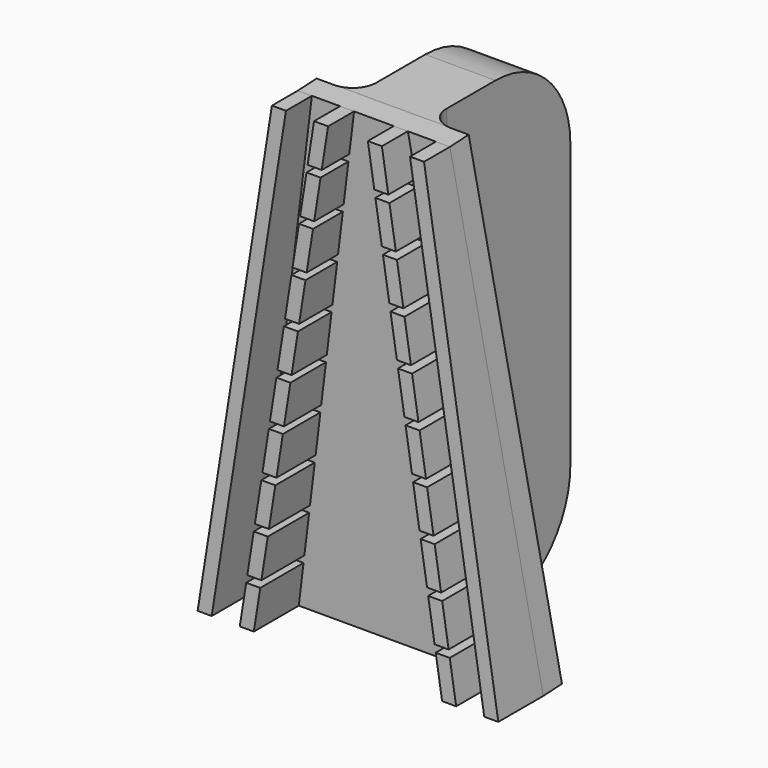
from build123d import *

# Parameters (mm, degrees)
F1_DEPTH     = 12
F3_DEPTH     = 40
F5_DEPTH     = 5
F6_W         = 38
F6_H         = 100.4237157875
F7_DEPTH     = 7.5
F9_DEPTH     = 7.5
F10_T4_DEPTH = 100.2951088773
F10_T9_DEPTH = 100.2951088773
F11_R        = 20


# Not quite as in the source:
# - a fillet or chamfer that OpenCascade refuses, or shapes differently, is made with other operations: its cross-section is extruded or revolved along the edge and cut away or added


with BuildPart() as f1:
    # F0 (on Front) → F1 (new body)
    with BuildSketch(Plane.XZ):
        Polygon((-18.7375766605, 8.6666666667), (-21.7375766605, 8.6666666667), (-23.11024181, 0), (-20.11024181, 0), align=None)
    extrude(amount=F1_DEPTH)


with BuildPart() as f1b:
    # F0 (on Front) → F1, piece 2 (new body)
    with BuildSketch(Plane.XZ):
        Polygon((21.7375766605, 8.6666666667), (18.7375766605, 8.6666666667), (20.11024181, 0), (23.11024181, 0), align=None)
    extrude(amount=F1_DEPTH)


with BuildPart() as f1c:
    # F0 (on Front) → F1, piece 3 (new body)
    with BuildSketch(Plane.XZ):
        Polygon((-20.1273348505, 18.8333333333), (-21.5, 10.1666666667), (-18.5, 10.1666666667), (-17.1273348505, 18.8333333333), align=None)
    extrude(amount=F1_DEPTH)


with BuildPart() as f1d:
    # F0 (on Front) → F1, piece 4 (new body)
    with BuildSketch(Plane.XZ):
        Polygon((17.1273348505, 18.8333333333), (18.5, 10.1666666667), (21.5, 10.1666666667), (20.1273348505, 18.8333333333), align=None)
    extrude(amount=F1_DEPTH)


with BuildPart() as f1e:
    # F0 (on Front) → F1, piece 5 (new body)
    with BuildSketch(Plane.XZ):
        Polygon((-15.5170930406, 29), (-18.5170930406, 29), (-19.88975819, 20.3333333333), (-16.88975819, 20.3333333333), align=None)
    extrude(amount=F1_DEPTH)


with BuildPart() as f1f:
    # F0 (on Front) → F1, piece 6 (new body)
    with BuildSketch(Plane.XZ):
        Polygon((16.88975819, 20.3333333333), (19.88975819, 20.3333333333), (18.5170930406, 29), (15.5170930406, 29), align=None)
    extrude(amount=F1_DEPTH)


with BuildPart() as f1g:
    # F0 (on Front) → F1, piece 7 (new body)
    with BuildSketch(Plane.XZ):
        Polygon((-15.2966094206, 49.3333333333), (-16.6692745701, 40.6666666667), (-13.6692745701, 40.6666666667), (-12.2966094206, 49.3333333333), align=None)
    extrude(amount=F1_DEPTH)


with BuildPart() as f1h:
    # F0 (on Front) → F1, piece 8 (new body)
    with BuildSketch(Plane.XZ):
        Polygon((-10.6863676107, 59.5), (-13.6863676107, 59.5), (-15.0590327601, 50.8333333333), (-12.0590327601, 50.8333333333), align=None)
    extrude(amount=F1_DEPTH)


with BuildPart() as f1i:
    # F0 (on Front) → F1, piece 9 (new body)
    with BuildSketch(Plane.XZ):
        Polygon((-11.8385491402, 71.1666666667), (-8.8385491402, 71.1666666667), (-7.4658839907, 79.8333333333), (-10.4658839907, 79.8333333333), align=None)
    extrude(amount=F1_DEPTH)


with BuildPart() as f1j:
    # F0 (on Front) → F1, piece 10 (new body)
    with BuildSketch(Plane.XZ):
        Polygon((-5.8556421808, 90), (-8.8556421808, 90), (-10.2283073302, 81.3333333333), (-7.2283073302, 81.3333333333), align=None)
    extrude(amount=F1_DEPTH)


with BuildPart() as f1k:
    # F0 (on Front) → F1, piece 11 (new body)
    with BuildSketch(Plane.XZ):
        Polygon((-4.2454003708, 100.1666666667), (-7.2454003708, 100.1666666667), (-8.6180655203, 91.5), (-5.6180655203, 91.5), align=None)
    extrude(amount=F1_DEPTH)


with BuildPart() as f1l:
    # F0 (on Front) → F1, piece 12 (new body)
    with BuildSketch(Plane.XZ):
        Polygon((16.9068512306, 39.1666666667), (13.9068512306, 39.1666666667), (15.2795163801, 30.5), (18.2795163801, 30.5), align=None)
    extrude(amount=F1_DEPTH)


with BuildPart() as f1m:
    # F0 (on Front) → F1, piece 13 (new body)
    with BuildSketch(Plane.XZ):
        Polygon((15.2966094206, 49.3333333333), (12.2966094206, 49.3333333333), (13.6692745701, 40.6666666667), (16.6692745701, 40.6666666667), align=None)
    extrude(amount=F1_DEPTH)


with BuildPart() as f1n:
    # F0 (on Front) → F1, piece 14 (new body)
    with BuildSketch(Plane.XZ):
        Polygon((13.6863676107, 59.5), (10.6863676107, 59.5), (12.0590327601, 50.8333333333), (15.0590327601, 50.8333333333), align=None)
    extrude(amount=F1_DEPTH)


with BuildPart() as f1o:
    # F0 (on Front) → F1, piece 15 (new body)
    with BuildSketch(Plane.XZ):
        Polygon((10.4487909502, 61), (13.4487909502, 61), (12.0761258007, 69.6666666667), (9.0761258007, 69.6666666667), align=None)
    extrude(amount=F1_DEPTH)


with BuildPart() as f1p:
    # F0 (on Front) → F1, piece 16 (new body)
    with BuildSketch(Plane.XZ):
        Polygon((10.4658839907, 79.8333333333), (7.4658839907, 79.8333333333), (8.8385491402, 71.1666666667), (11.8385491402, 71.1666666667), align=None)
    extrude(amount=F1_DEPTH)


with BuildPart() as f1q:
    # F0 (on Front) → F1, piece 17 (new body)
    with BuildSketch(Plane.XZ):
        Polygon((8.8556421808, 90), (5.8556421808, 90), (7.2283073302, 81.3333333333), (10.2283073302, 81.3333333333), align=None)
    extrude(amount=F1_DEPTH)


with BuildPart() as f1r:
    # F0 (on Front) → F1, piece 18 (new body)
    with BuildSketch(Plane.XZ):
        Polygon((-13.9068512306, 39.1666666667), (-16.9068512306, 39.1666666667), (-18.2795163801, 30.5), (-15.2795163801, 30.5), align=None)
    extrude(amount=F1_DEPTH)


with BuildPart() as f1s:
    # F0 (on Front) → F1, piece 19 (new body)
    with BuildSketch(Plane.XZ):
        Polygon((-12.0761258007, 69.6666666667), (-13.4487909502, 61), (-10.4487909502, 61), (-9.0761258007, 69.6666666667), align=None)
    extrude(amount=F1_DEPTH)


with BuildPart() as f1t:
    # F0 (on Front) → F1, piece 20 (new body)
    with BuildSketch(Plane.XZ):
        Polygon((7.2454003708, 100.1666666667), (4.2454003708, 100.1666666667), (5.6180655203, 91.5), (8.6180655203, 91.5), align=None)
    extrude(amount=F1_DEPTH)


with BuildPart() as f1u:
    # F0 (on Front) → F1, piece 21 (new body)
    with BuildSketch(Plane.XZ):
        Polygon((-29.11024181, 0), (-13.2454003708, 100.1666666667), (-16.2454003708, 100.1666666667), (-32.11024181, 0), align=None)
    extrude(amount=F1_DEPTH)


with BuildPart() as f1v:
    # F0 (on Front) → F1, piece 22 (new body)
    with BuildSketch(Plane.XZ):
        Polygon((16.2454003708, 100.1666666667), (13.2454003708, 100.1666666667), (29.11024181, 0), (32.11024181, 0), align=None)
    extrude(amount=F1_DEPTH)


with BuildPart() as f3_tool:
    # F2 (on Right) → F3 (new body, symmetric)
    with BuildSketch(Plane.YZ):
        Polygon((-5.0742244334, 100.1666666667), (0, 0), (0, 100.1666666667), align=None)
    extrude(amount=F3_DEPTH, both=True)


with BuildPart() as f1_1:
    add(f1.part)

    # F3: cut by f3_tool
    add(f3_tool.part, mode=Mode.SUBTRACT)



with BuildPart() as f1b_1:
    add(f1b.part)

    # F3: cut by f3_tool
    add(f3_tool.part, mode=Mode.SUBTRACT)


with BuildPart() as f1c_1:
    add(f1c.part)

    # F3: cut by f3_tool
    add(f3_tool.part, mode=Mode.SUBTRACT)


with BuildPart() as f1d_1:
    add(f1d.part)

    # F3: cut by f3_tool
    add(f3_tool.part, mode=Mode.SUBTRACT)


with BuildPart() as f1e_1:
    add(f1e.part)

    # F3: cut by f3_tool
    add(f3_tool.part, mode=Mode.SUBTRACT)


with BuildPart() as f1f_1:
    add(f1f.part)

    # F3: cut by f3_tool
    add(f3_tool.part, mode=Mode.SUBTRACT)


with BuildPart() as f1g_1:
    add(f1g.part)

    # F3: cut by f3_tool
    add(f3_tool.part, mode=Mode.SUBTRACT)


with BuildPart() as f1h_1:
    add(f1h.part)

    # F3: cut by f3_tool
    add(f3_tool.part, mode=Mode.SUBTRACT)


with BuildPart() as f1i_1:
    add(f1i.part)

    # F3: cut by f3_tool
    add(f3_tool.part, mode=Mode.SUBTRACT)


with BuildPart() as f1j_1:
    add(f1j.part)

    # F3: cut by f3_tool
    add(f3_tool.part, mode=Mode.SUBTRACT)


with BuildPart() as f1k_1:
    add(f1k.part)

    # F3: cut by f3_tool
    add(f3_tool.part, mode=Mode.SUBTRACT)


with BuildPart() as f1l_1:
    add(f1l.part)

    # F3: cut by f3_tool
    add(f3_tool.part, mode=Mode.SUBTRACT)


with BuildPart() as f1m_1:
    add(f1m.part)

    # F3: cut by f3_tool
    add(f3_tool.part, mode=Mode.SUBTRACT)


with BuildPart() as f1n_1:
    add(f1n.part)

    # F3: cut by f3_tool
    add(f3_tool.part, mode=Mode.SUBTRACT)


with BuildPart() as f1o_1:
    add(f1o.part)

    # F3: cut by f3_tool
    add(f3_tool.part, mode=Mode.SUBTRACT)


with BuildPart() as f1p_1:
    add(f1p.part)

    # F3: cut by f3_tool
    add(f3_tool.part, mode=Mode.SUBTRACT)


with BuildPart() as f1q_1:
    add(f1q.part)

    # F3: cut by f3_tool
    add(f3_tool.part, mode=Mode.SUBTRACT)


with BuildPart() as f1r_1:
    add(f1r.part)

    # F3: cut by f3_tool
    add(f3_tool.part, mode=Mode.SUBTRACT)


with BuildPart() as f1s_1:
    add(f1s.part)

    # F3: cut by f3_tool
    add(f3_tool.part, mode=Mode.SUBTRACT)


with BuildPart() as f1t_1:
    add(f1t.part)

    # F3: cut by f3_tool
    add(f3_tool.part, mode=Mode.SUBTRACT)


with BuildPart() as f1u_1:
    add(f1u.part)

    # F3: cut by f3_tool
    add(f3_tool.part, mode=Mode.SUBTRACT)


with BuildPart() as f1v_1:
    add(f1v.part)

    # F3: cut by f3_tool
    add(f3_tool.part, mode=Mode.SUBTRACT)


with BuildPart() as f1_2:
    add(f1_1.part)

    add(f1b_1.part)  # F5 merges F1b

    add(f1c_1.part)  # F5 merges F1c

    add(f1d_1.part)  # F5 merges F1d

    add(f1e_1.part)  # F5 merges F1e

    add(f1f_1.part)  # F5 merges F1f

    add(f1g_1.part)  # F5 merges F1g

    add(f1h_1.part)  # F5 merges F1h

    add(f1i_1.part)  # F5 merges F1i

    add(f1j_1.part)  # F5 merges F1j

    add(f1k_1.part)  # F5 merges F1k

    add(f1l_1.part)  # F5 merges F1l

    add(f1m_1.part)  # F5 merges F1m

    add(f1n_1.part)  # F5 merges F1n

    add(f1o_1.part)  # F5 merges F1o

    add(f1p_1.part)  # F5 merges F1p

    add(f1q_1.part)  # F5 merges F1q

    add(f1r_1.part)  # F5 merges F1r

    add(f1s_1.part)  # F5 merges F1s

    add(f1t_1.part)  # F5 merges F1t

    add(f1u_1.part)  # F5 merges F1u

    add(f1v_1.part)  # F5 merges F1v
    # F4 (on face) → F5 (join)
    with BuildSketch(Plane(origin=(0, 0, 0), x_dir=(-1, 0, 0), z_dir=(0, 0.9987193572, 0.0505929401))):
        Polygon((16.2454003708, 100.2951088773), (-16.2454003708, 100.2951088773), (-32.11024181, 0), (32.11024181, 0), align=None)
    extrude(amount=F5_DEPTH)

    # F6 (on Right) → F7 (join, symmetric)
    with BuildSketch(Plane.YZ):
        with Locations((19, 50.2118578937)):
            Rectangle(F6_W, F6_H)
    extrude(amount=F7_DEPTH, both=True)

    # F8 (on Right) → F9 (join, symmetric)
    with BuildSketch(Plane.YZ):
        Polygon((0.7220453882, 99.8437014869), (0, 100.4237157875), (-0.0806276475, 100.4196313671), (-0.4271789039, 99.9818352512), (-0.1710176838, 98.3370152763), align=None)
    extrude(amount=F9_DEPTH, both=True)

    # F10: fillet of radius 5 on 2 edges, made by hand


with BuildPart() as f10_tool2:
    # F10_s3 → F10_t4 (new body)
    with BuildSketch(Plane(origin=(0, 0, 0), x_dir=(1, 0, 0), z_dir=(0, -0.0505929401, 0.9987193572))):
        with BuildLine():
            ThreePointArc((12.5, 5), (8.9644660941, 6.4644660941), (7.5, 10))
            Line((7.5, 10), (7.5, 5))
            Line((7.5, 5), (12.5, 5))
        make_face()
    extrude(amount=F10_T4_DEPTH)

    split(bisect_by=Plane.XY.offset(100.4237157875), keep=Keep.BOTTOM)


with BuildPart() as f1_3:
    add(f1_2.part)

    # F10_t1: union F10_tool2
    add(f10_tool2.part)


with BuildPart() as f10_tool7:
    # F10_s8 → F10_t9 (new body)
    with BuildSketch(Plane(origin=(0, -5.0742244334, 100.1666666667), x_dir=(1, 0, 0), z_dir=(0, 0.0505929401, -0.9987193572))):
        with BuildLine():
            ThreePointArc((-7.5, -10), (-8.9644660941, -6.4644660941), (-12.5, -5))
            Line((-12.5, -5), (-7.5, -5))
            Line((-7.5, -5), (-7.5, -10))
        make_face()
    extrude(amount=F10_T9_DEPTH)

    split(bisect_by=Plane.XY.offset(100.4237157875), keep=Keep.BOTTOM)


with BuildPart() as f1_4:
    add(f1_3.part)

    # F10_t6: union F10_tool7
    add(f10_tool7.part)

    # F11
    f11_edges = [f1_4.edges().sort_by_distance(p)[0] for p in [
        (0, 38, 100.423716),
        (0, 38, 0),
    ]]
    fillet(f11_edges, radius=F11_R)


solid = f1_4.part
